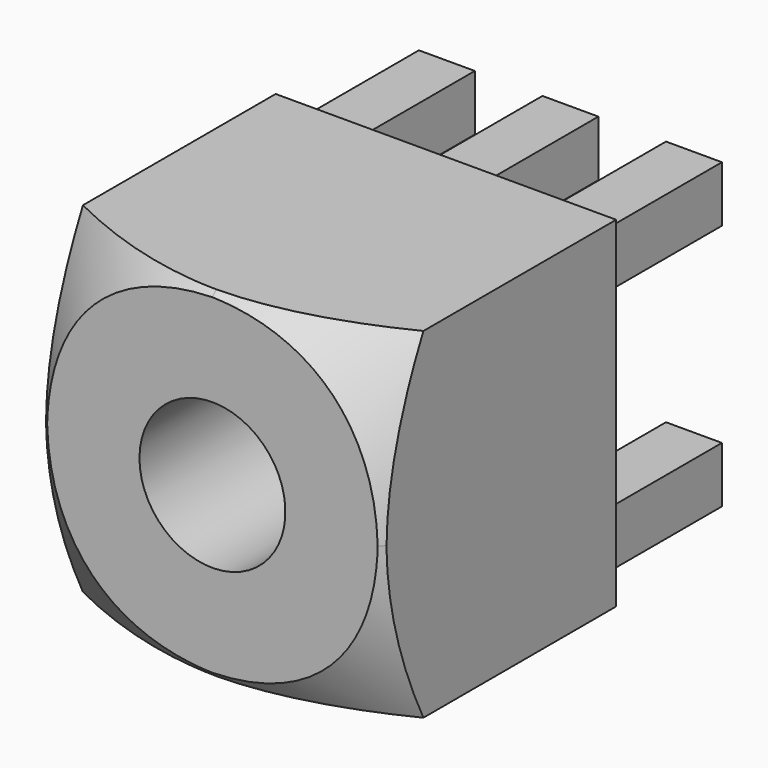
from build123d import *

# Parameters (mm, degrees)
F0_W        = 7
F0_H        = 7
F0_W_2      = 1.15
F0_H_2      = 1.15
F1_DEPTH    = 6
F2_SIZE     = 0.1
F3_T1_DEPTH = 14.6069618105
F3_T3_DEPTH = 14.6069618105
F3_T5_DEPTH = 14.6069618105
F3_T7_DEPTH = 14.6069618105
F6_D        = 3
F6_DEPTH    = 6
F6_TIP      = 0.9012909285
F8_DEPTH    = 3.5
F9_SIZE     = 0.3


# Not quite as in the source:
# - a fillet or chamfer that OpenCascade refuses, or shapes differently, is made with other operations: its cross-section is extruded or revolved along the edge and cut away or added


with BuildPart() as f1:
    # F0 (on Front) → F1 (new body)
    with BuildSketch(Plane.XZ):
        Rectangle(F0_W, F0_H)
        with Locations((-2.54, -2.54)):
            Rectangle(F0_W_2, F0_H_2, mode=Mode.SUBTRACT)
        with Locations((0, -2.54)):
            Rectangle(F0_W_2, F0_H_2, mode=Mode.SUBTRACT)
        with Locations((2.54, -2.54)):
            Rectangle(F0_W_2, F0_H_2, mode=Mode.SUBTRACT)
        with Locations((-2.54, 2.54)):
            Rectangle(F0_W_2, F0_H_2, mode=Mode.SUBTRACT)
        with Locations((0, 2.54)):
            Rectangle(F0_W_2, F0_H_2, mode=Mode.SUBTRACT)
        with Locations((2.54, 2.54)):
            Rectangle(F0_W_2, F0_H_2, mode=Mode.SUBTRACT)
        with Locations((-2.54, -2.54)):
            Rectangle(F0_W_2, F0_H_2)
        with Locations((0, -2.54)):
            Rectangle(F0_W_2, F0_H_2)
        with Locations((0, 2.54)):
            Rectangle(F0_W_2, F0_H_2)
        with Locations((-2.54, 2.54)):
            Rectangle(F0_W_2, F0_H_2)
        with Locations((2.54, 2.54)):
            Rectangle(F0_W_2, F0_H_2)
        with Locations((2.54, -2.54)):
            Rectangle(F0_W_2, F0_H_2)
    extrude(amount=F1_DEPTH)

    # F2
    f2_edges = [f1.edges().sort_by_distance(p)[0] for p in [
        (3.5, -6, 0),
        (0, -6, 3.5),
        (-3.5, -6, 0),
        (0, -6, -3.5),
    ]]
    chamfer(f2_edges, length=F2_SIZE)

    # F3: fillet of radius 5 on 4 edges, made by hand

    # F3_s2 → F3_t1 (cut)
    with BuildSketch(Plane(origin=(4.5333333333, 4.5333333333, 4.5333333333), x_dir=(0.7071067812, -0.7071067812, 0), z_dir=(-0.5773502692, -0.5773502692, -0.5773502692))):
        with BuildLine():
            ThreePointArc((4.1468037432, 5.2809096033), (5.9769307621, 3.4507825844), (6.6468037432, 0.9507825844))
            Line((6.6468037432, 0.9507825844), (6.6468037432, 3.8375339304))
            Line((6.6468037432, 3.8375339304), (4.1468037432, 5.2809096033))
        make_face()
    extrude(amount=F3_T1_DEPTH, mode=Mode.SUBTRACT)

    # F3_s4 → F3_t3 (cut)
    with BuildSketch(Plane(origin=(-4.5333333333, 4.5333333333, 4.5333333333), x_dir=(0.7071067812, 0.7071067812, 0), z_dir=(0.5773502692, -0.5773502692, -0.5773502692))):
        with BuildLine():
            ThreePointArc((-4.1468037432, 5.2809096033), (-5.9769307621, 3.4507825844), (-6.6468037432, 0.9507825844))
            Line((-6.6468037432, 0.9507825844), (-6.6468037432, 3.8375339304))
            Line((-6.6468037432, 3.8375339304), (-4.1468037432, 5.2809096033))
        make_face()
    extrude(amount=F3_T3_DEPTH, mode=Mode.SUBTRACT)

    # F3_s6 → F3_t5 (cut)
    with BuildSketch(Plane(origin=(4.5333333333, 4.5333333333, -4.5333333333), x_dir=(0.7071067812, -0.7071067812, 0), z_dir=(-0.5773502692, -0.5773502692, 0.5773502692))):
        with BuildLine():
            ThreePointArc((6.6468037432, -0.9507825844), (5.9769307621, -3.4507825844), (4.1468037432, -5.2809096033))
            Line((4.1468037432, -5.2809096033), (6.6468037432, -3.8375339304))
            Line((6.6468037432, -3.8375339304), (6.6468037432, -0.9507825844))
        make_face()
    extrude(amount=F3_T5_DEPTH, mode=Mode.SUBTRACT)

    # F3_s8 → F3_t7 (cut)
    with BuildSketch(Plane(origin=(-4.5333333333, 4.5333333333, -4.5333333333), x_dir=(0.7071067812, 0.7071067812, 0), z_dir=(0.5773502692, -0.5773502692, 0.5773502692))):
        with BuildLine():
            ThreePointArc((-6.6468037432, -0.9507825844), (-5.9769307621, -3.4507825844), (-4.1468037432, -5.2809096033))
            Line((-4.1468037432, -5.2809096033), (-6.6468037432, -3.8375339304))
            Line((-6.6468037432, -3.8375339304), (-6.6468037432, -0.9507825844))
        make_face()
    extrude(amount=F3_T7_DEPTH, mode=Mode.SUBTRACT)

    # F6
    with Locations(Plane.XZ.offset(6)):
        with Locations((0, 0)):
            Hole(F6_D / 2, depth=F6_DEPTH)
            with Locations((0, 0, -(F6_DEPTH + F6_TIP / 2))):  # 118° drill point
                Cone(0, F6_D / 2, F6_TIP, mode=Mode.SUBTRACT)

    # F0 (on Front) → F8 (join)
    with BuildSketch(Plane.XZ):
        with Locations((2.54, 2.54)):
            Rectangle(F0_W_2, F0_H_2)
        with Locations((0, 2.54)):
            Rectangle(F0_W_2, F0_H_2)
        with Locations((-2.54, 2.54)):
            Rectangle(F0_W_2, F0_H_2)
        with Locations((-2.54, -2.54)):
            Rectangle(F0_W_2, F0_H_2)
        with Locations((0, -2.54)):
            Rectangle(F0_W_2, F0_H_2)
        with Locations((2.54, -2.54)):
            Rectangle(F0_W_2, F0_H_2)
    extrude(amount=-F8_DEPTH)

    # F9
    f9_edges = [f1.edges().sort_by_distance(p)[0] for p in [
        (2.54, 3.5, -3.115),
        (1.965, 3.5, -2.54),
        (3.115, 3.5, -2.54),
        (2.54, 3.5, -1.965),
        (0.575, 3.5, -2.54),
        (0, 3.5, -3.115),
        (-0.575, 3.5, -2.54),
        (0, 3.5, -1.965),
        (-1.965, 3.5, -2.54),
        (-2.54, 3.5, -1.965),
        (-3.115, 3.5, -2.54),
        (-2.54, 3.5, -3.115),
        (3.115, 3.5, 2.54),
        (2.54, 3.5, 1.965),
        (1.965, 3.5, 2.54),
        (2.54, 3.5, 3.115),
        (0.575, 3.5, 2.54),
        (0, 3.5, 3.115),
        (-0.575, 3.5, 2.54),
        (0, 3.5, 1.965),
        (-1.965, 3.5, 2.54),
        (-2.54, 3.5, 1.965),
        (-3.115, 3.5, 2.54),
        (-2.54, 3.5, 3.115),
    ]]
    chamfer(f9_edges, length=F9_SIZE)


solid = f1.part
